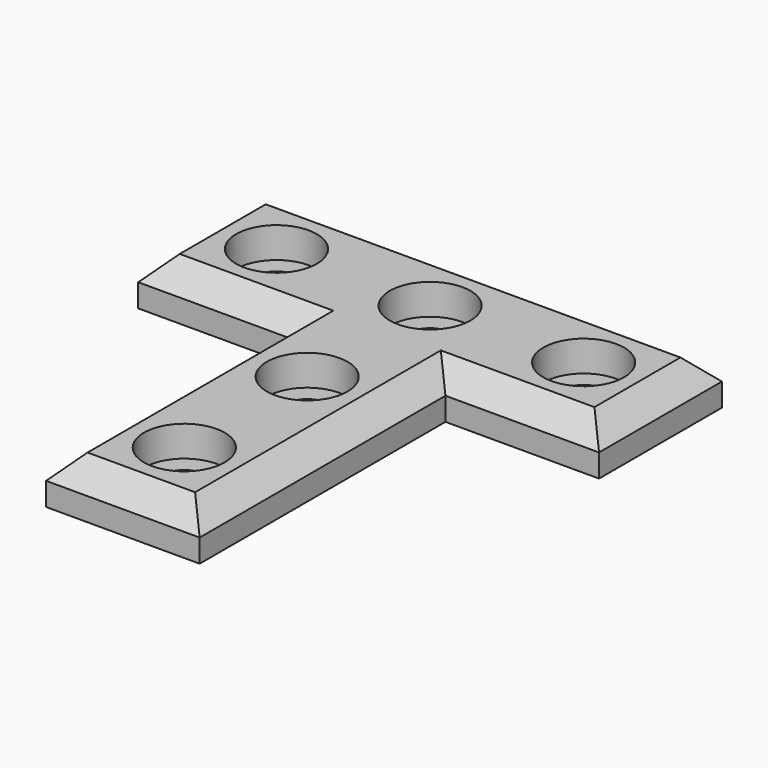
from build123d import *

# Parameters (mm, degrees)
F2_R     = 2.75
F3_DEPTH = 6
F4_SIZE  = 3
F5_R     = 5.25
F5_R_2   = 2.75
F6_DEPTH = 4


with BuildPart() as f3:
    # F2 (on Top) → F3 (new body)
    with BuildSketch(Plane.XY):
        Polygon((-10, -50), (0, -50), (10, -50), (10, -10), (30, -10), (30, 10), (0, 10), (-30, 10), (-30, -10), (-10, -10), align=None)
        with Locations((0, -40)):
            Circle(F2_R, mode=Mode.SUBTRACT)
        with Locations((-20, 0)):
            Circle(F2_R, mode=Mode.SUBTRACT)
        with Locations((0, -20)):
            Circle(F2_R, mode=Mode.SUBTRACT)
        Circle(F2_R, mode=Mode.SUBTRACT)
        with Locations((20, 0)):
            Circle(F2_R, mode=Mode.SUBTRACT)
    extrude(amount=F3_DEPTH)

    # F4
    f4_edges = [f3.edges().sort_by_distance(p)[0] for p in [
        (0, -50, 6),
        (10, -30, 6),
        (20, -10, 6),
        (30, 0, 6),
        (0, 10, 6),
        (-30, 0, 6),
        (-20, -10, 6),
        (-10, -30, 6),
    ]]
    chamfer(f4_edges, length=F4_SIZE)

    # F5 (on face) → F6 (cut)
    with BuildSketch(Plane.XY.offset(6)):
        with Locations((-20, 0)):
            Circle(F5_R)
        with Locations((-20, 0)):
            Circle(F5_R_2, mode=Mode.SUBTRACT)
        Circle(F5_R)
        Circle(F5_R_2, mode=Mode.SUBTRACT)
        with Locations((20, 0)):
            Circle(F5_R)
        with Locations((20, 0)):
            Circle(F5_R_2, mode=Mode.SUBTRACT)
        with Locations((0, -20)):
            Circle(F5_R)
        with Locations((0, -20)):
            Circle(F5_R_2, mode=Mode.SUBTRACT)
        with Locations((0, -40)):
            Circle(F5_R)
        with Locations((0, -40)):
            Circle(F5_R_2, mode=Mode.SUBTRACT)
    extrude(amount=-F6_DEPTH, mode=Mode.SUBTRACT)


solid = f3.part
